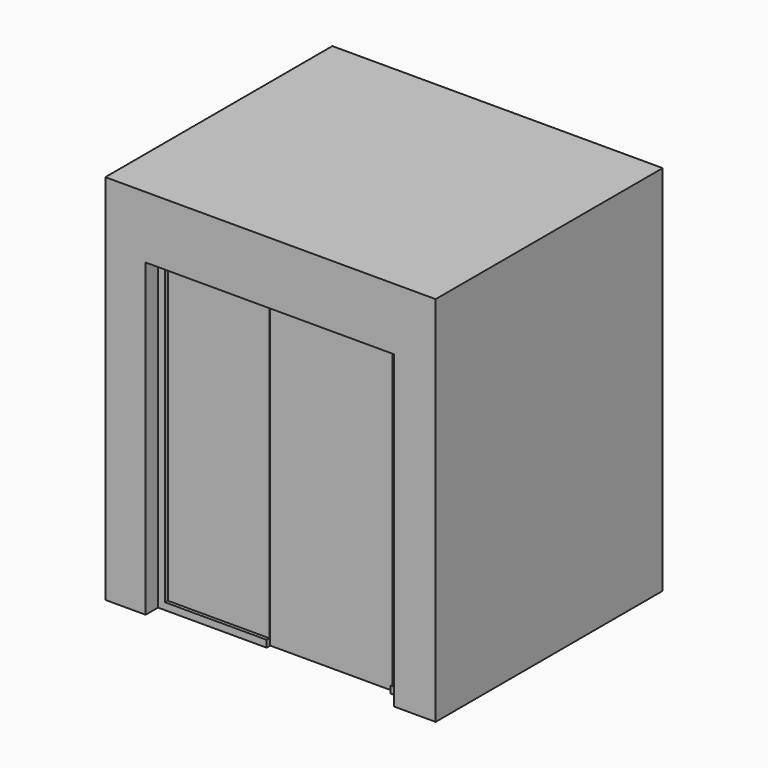
from build123d import *

# Parameters (mm, degrees)
F0_W      = 2130
F0_H      = 1830
F0_W_2    = 1800
F0_H_2    = 1500
F1_DEPTH  = 2400
F2_W      = 1600
F2_H      = 2000
F3_DEPTH  = 165
F4_W      = 2130
F4_H      = 1830
F5_DEPTH  = 400
F8_DEPTH  = 50
F10_W     = 695
F10_H     = 1990
F11_DEPTH = 3
F10_W_2   = 790
F10_W_3   = 95
F12_W     = 540
F12_H     = 28
F13_DEPTH = 1800
F14_W     = 1800
F14_H     = 478
F15_DEPTH = 28
F16_W     = 1800
F16_H     = 28
F17_DEPTH = 460
F18_W     = 1800
F18_H     = 95
F19_DEPTH = 28
F21_DEPTH = 1300


with BuildPart() as f1:
    # F0 (on Top) → F1 (new body)
    with BuildSketch(Plane.XY):
        with Locations((900, -750)):
            Rectangle(F0_W, F0_H)
        with Locations((900, -750)):
            Rectangle(F0_W_2, F0_H_2, mode=Mode.SUBTRACT)
    extrude(amount=F1_DEPTH)

    # F2 (on face) → F3 (cut, through all)
    with BuildSketch(Plane.XZ.offset(1665)):
        with Locations((895, 1000)):
            Rectangle(F2_W, F2_H)
    extrude(amount=-F3_DEPTH, mode=Mode.SUBTRACT)

    # F4 (on face) → F5 (join, through all)
    with BuildSketch(Plane.XY.offset(2400)):
        with Locations((900, -750)):
            Rectangle(F4_W, F4_H)
    extrude(amount=-F5_DEPTH)


with BuildPart() as f8:
    # F7 (on offset) → F8 (new body)
    with BuildSketch(Plane.XZ.offset(1565)):
        Polygon((795, 45), (140, 45), (140, 1955), (795, 1955), (795, 2000), (95, 2000), (95, 0), (795, 0), align=None)
    extrude(amount=-F8_DEPTH)


with BuildPart() as f8b:
    # F7 (on offset) → F8, piece 2 (new body)
    with BuildSketch(Plane.XZ.offset(1565)):
        Polygon((1595, 1955), (1650, 1955), (1650, 45), (1595, 45), (1595, 0), (1695, 0), (1695, 2000), (1595, 2000), align=None)
    extrude(amount=-F8_DEPTH)


with BuildPart() as f11:
    # F10 (on offset) → F11 (new body, symmetric)
    with BuildSketch(Plane.XZ.offset(1540)):
        with Locations((447.5, 1000)):
            Rectangle(F10_W, F10_H)
    extrude(amount=F11_DEPTH, both=True)


with BuildPart() as f11b:
    # F10 (on offset) → F11, piece 2 (new body, symmetric)
    with BuildSketch(Plane.XZ.offset(1540)):
        with Locations((1195, 1000)):
            Rectangle(F10_W_2, F10_H)
    extrude(amount=F11_DEPTH, both=True)


with BuildPart() as f11c:
    # F10 (on offset) → F11, piece 3 (new body, symmetric)
    with BuildSketch(Plane.XZ.offset(1540)):
        with Locations((1642.5, 1000)):
            Rectangle(F10_W_3, F10_H)
    extrude(amount=F11_DEPTH, both=True)


with BuildPart() as f13:
    # F12 (on face) → F13 (new body, through all)
    with BuildSketch(Plane(origin=(1800, 0, 0), x_dir=(0, -1, 0), z_dir=(-1, 0, 0))):
        with Locations((270, 926)):
            Rectangle(F12_W, F12_H)
    extrude(amount=F13_DEPTH)

    # F14 (on face) → F15 (join)
    with BuildSketch(Plane.XZ.offset(540)):
        with Locations((900, 701)):
            Rectangle(F14_W, F14_H)
    extrude(amount=-F15_DEPTH)

    # F16 (on face) → F17 (join)
    with BuildSketch(Plane.XZ.offset(540)):
        with Locations((900, 476)):
            Rectangle(F16_W, F16_H)
    extrude(amount=F17_DEPTH)

    # F18 (on face) → F19 (join)
    with BuildSketch(Plane.XZ.offset(1000)):
        with Locations((900, 442.5)):
            Rectangle(F18_W, F18_H)
    extrude(amount=-F19_DEPTH)


with BuildPart() as f21:
    # F20 (on face) → F21 (new body)
    with BuildSketch(Plane(origin=(0, 0, 0), x_dir=(1, 0, 0), z_dir=(0, 0, -1))):
        with BuildLine():
            Line((30, 1442.5), (30, 1057.5))
            ThreePointArc((30, 1057.5), (250, 1250), (30, 1442.5))
        make_face()
    extrude(amount=-F21_DEPTH)


solid = Compound([f1.part, f8.part, f8b.part, f11.part, f11b.part, f11c.part, f13.part, f21.part])
